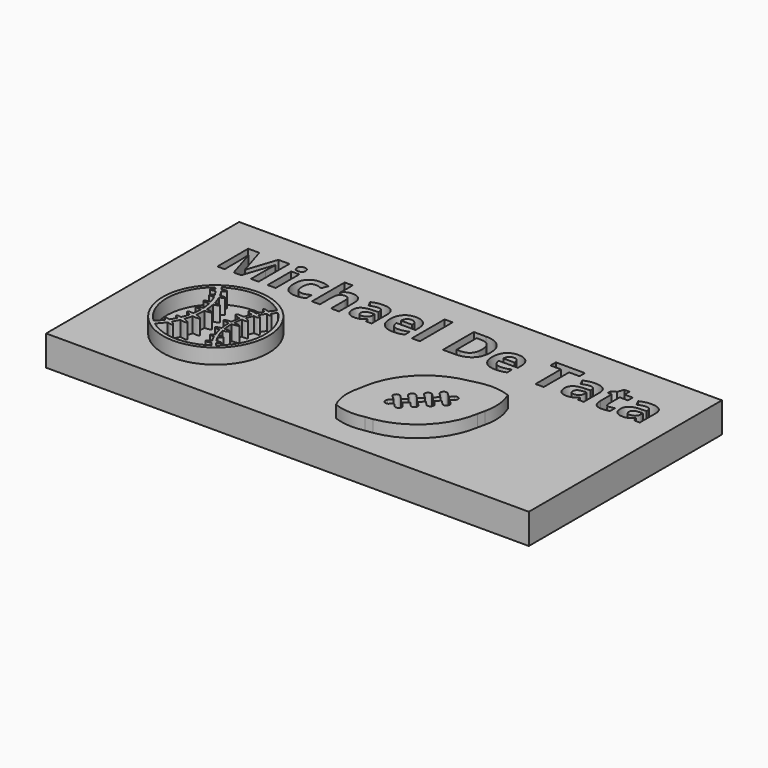
from build123d import *

# Parameters (mm, degrees)
F0_W         = 101.6
F0_H         = 50.8
F1_DEPTH     = 6.35
F3_R         = 11.1218952469
F4_DEPTH     = 3.175
F6_DEPTH     = 2.54
F2_TEXT_SIZE = 11.3601718719
F7_DEPTH     = 3.175


# Not quite as in the source:
# - a feature names something its author has since deleted; it is built from what else it names
# - Text() gives the source's letters only with a copy of the font that has no kerning and outlines rounded to 1/6400 em; it was checked with that copy


with BuildPart() as f1:
    # F0 (on Top) → F1 (new body)
    with BuildSketch(Plane.XY):
        Rectangle(F0_W, F0_H)
    extrude(amount=F1_DEPTH)

    # F3 (on face) → F4 (join)
    with BuildSketch(Plane.XY.offset(6.35)):
        with Locations((-29.0186479688, -7.998152636)):
            Circle(F3_R)
        with BuildLine():
            ThreePointArc((-22.6005740509, -1.5785002837), (-22.1799453907, -1.1150611958), (-21.7337125174, -0.6762212695))
            ThreePointArc((-21.7337125174, -0.6762212695), (-18.7036022056, -8.5280529742), (-22.5223602891, -16.0280473955))
            ThreePointArc((-22.5223602891, -16.0280473955), (-22.7780684113, -15.7253880437), (-23.0227432081, -15.4137414958))
            add(Edge.make_bspline(
                [(-23.0227432081, -15.4137414958), (-19.8096573759, -13.5154492667), (-23.4284209645, -14.8404104762)],
                knots=[5.0949228166, 5.0949228166, 5.0949228166, 7.5723181465, 7.5723181465, 7.5723181465], degree=2, weights=[1, 0.3260277363, 1]))
            ThreePointArc((-23.4284209645, -14.8404104762), (-23.805157256, -14.2278051435), (-24.1411783748, -13.5919550552))
            add(Edge.make_bspline(
                [(-24.1411783748, -13.5919550552), (-23.230493802, -13.2932672954), (-23.3456804393, -13.0374149632), (-23.4608670766, -12.7815626311), (-24.417649348, -12.9778582733)],
                knots=[4.9642155268, 4.9642155268, 4.9642155268, 6.3335518412, 6.3335518412, 7.7028881555, 7.7028881555, 7.7028881555], degree=2, weights=[1, 0.7746289525, 1, 0.7746289525, 1]))
            ThreePointArc((-24.417649348, -12.9778582733), (-24.7272451793, -12.1343360676), (-24.9671670987, -11.2684164623))
            add(Edge.make_bspline(
                [(-24.9671670987, -11.2684164623), (-23.7185142099, -11.0757901304), (-23.7819942791, -10.7558740683), (-23.8454743483, -10.4359580061), (-25.1117428322, -10.5398082556)],
                knots=[4.8729813766, 4.8729813766, 4.8729813766, 6.3045795957, 6.3045795957, 7.7361778148, 7.7361778148, 7.7361778148], degree=2, weights=[1, 0.75456909, 1, 0.75456909, 1]))
            ThreePointArc((-25.1117428322, -10.5398082556), (-25.2292975786, -9.5332747384), (-25.2539958206, -8.5202007843))
            add(Edge.make_bspline(
                [(-25.2539958206, -8.5202007843), (-23.9044438188, -8.4744131194), (-23.8901319743, -8.1956421106), (-23.8758201297, -7.9168711017), (-25.2203758909, -7.8653402803)],
                knots=[4.8773757852, 4.8773757852, 4.8773757852, 6.2727242396, 6.2727242396, 7.6680726941, 7.6680726941, 7.6680726941], degree=2, weights=[1, 0.7663384213, 1, 0.7663384213, 1]))
            ThreePointArc((-25.2203758909, -7.8653402803), (-25.1208078752, -7.0327925831), (-24.9582957446, -6.2102117269))
            add(Edge.make_bspline(
                [(-24.9582957446, -6.2102117269), (-20.6595931309, -6.796804342), (-24.7459385815, -5.4406721979)],
                knots=[5.0315591498, 5.0315591498, 5.0315591498, 7.5106380767, 7.5106380767, 7.5106380767], degree=2, weights=[1, 0.3252318181, 1]))
            ThreePointArc((-24.7459385815, -5.4406721979), (-24.4822237672, -4.6979294002), (-24.1661512275, -3.9759110372))
            add(Edge.make_bspline(
                [(-24.1661512275, -3.9759110372), (-20.9222938258, -4.6172431349), (-23.7986605821, -3.2771255195)],
                knots=[5.0646772946, 5.0646772946, 5.0646772946, 7.3959785173, 7.3959785173, 7.3959785173], degree=2, weights=[1, 0.3941526836, 1]))
            ThreePointArc((-23.7986605821, -3.2771255195), (-23.4215564836, -2.6655092164), (-23.0054379696, -2.0797384545))
            add(Edge.make_bspline(
                [(-23.0054379696, -2.0797384545), (-20.3352108354, -2.919747127), (-22.6005740509, -1.5785002837)],
                knots=[5.0589564234, 5.0589564234, 5.0589564234, 7.3589787004, 7.3589787004, 7.3589787004], degree=2, weights=[1, 0.408477274, 1]))
        make_face(mode=Mode.SUBTRACT)
        with BuildLine():
            ThreePointArc((-36.0519275049, -15.5621424847), (-39.3420122611, -7.6678298334), (-35.5539764132, 0))
            ThreePointArc((-35.5539764132, 0), (-35.35460765, -0.2062619443), (-35.1608345722, -0.4177894547))
            add(Edge.make_bspline(
                [(-35.1608345722, -0.4177894547), (-37.7982757436, -2.1762355745), (-34.7023311185, -0.9679386151)],
                knots=[2.0229375925, 2.0229375925, 2.0229375925, 4.3852414284, 4.3852414284, 4.3852414284], degree=2, weights=[1, 0.3798595016, 1]))
            ThreePointArc((-34.7023311185, -0.9679386151), (-34.2949359087, -1.527849727), (-33.9245732543, -2.1129162313))
            add(Edge.make_bspline(
                [(-33.9245732543, -2.1129162313), (-37.2277823305, -3.6536940562), (-33.5874672551, -2.7312571551)],
                knots=[1.9552328248, 1.9552328248, 1.9552328248, 4.4201232192, 4.4201232192, 4.4201232192], degree=2, weights=[1, 0.3319321592, 1]))
            ThreePointArc((-33.5874672551, -2.7312571551), (-33.2140250787, -3.5589351008), (-32.9120345986, -4.4152712444))
            add(Edge.make_bspline(
                [(-32.9120345986, -4.4152712444), (-34.1483285306, -4.6541693743), (-34.0707584589, -4.9420653759), (-33.9931883873, -5.2299613774), (-32.7256886081, -5.1068816097)],
                knots=[1.8023954855, 1.8023954855, 1.8023954855, 3.170663936, 3.170663936, 4.5389323865, 4.5389323865, 4.5389323865], degree=2, weights=[1, 0.7749665091, 1, 0.7749665091, 1]))
            ThreePointArc((-32.7256886081, -5.1068816097), (-32.5525243736, -6.0270238287), (-32.4603856609, -6.958773802))
            add(Edge.make_bspline(
                [(-32.4603856609, -6.958773802), (-33.8480769362, -7.0137831609), (-33.8414401354, -7.2896008469), (-33.8348033345, -7.5654185328), (-32.4445257743, -7.6178921517)],
                knots=[1.7715815328, 1.7715815328, 1.7715815328, 3.1462792098, 3.1462792098, 4.5209768868, 4.5209768868, 4.5209768868], degree=2, weights=[1, 0.7729308655, 1, 0.7729308655, 1]))
            ThreePointArc((-32.4445257743, -7.6178921517), (-32.488635289, -8.5195254569), (-32.6085160069, -9.4142415458))
            add(Edge.make_bspline(
                [(-32.6085160069, -9.4142415458), (-36.9972444639, -8.8518803338), (-32.7586754015, -10.1217847591)],
                knots=[1.9033850235, 1.9033850235, 1.9033850235, 4.379874232, 4.379874232, 4.379874232], degree=2, weights=[1, 0.3264560084, 1]))
            ThreePointArc((-32.7586754015, -10.1217847591), (-32.9938018326, -10.9324023236), (-33.2920310018, -11.721987428))
            add(Edge.make_bspline(
                [(-33.2920310018, -11.721987428), (-36.1690854529, -11.2401260388), (-33.5703416762, -12.3262507069)],
                knots=[1.9795308567, 1.9795308567, 1.9795308567, 4.2252146249, 4.2252146249, 4.2252146249], degree=2, weights=[1, 0.4331227092, 1]))
            ThreePointArc((-33.5703416762, -12.3262507069), (-33.9150089726, -12.9624918103), (-34.3018512886, -13.5740073942))
            add(Edge.make_bspline(
                [(-34.3018512886, -13.5740073942), (-36.7715845297, -12.7356918477), (-34.7165123024, -14.1419316901)],
                knots=[1.9598946097, 1.9598946097, 1.9598946097, 4.2150352925, 4.2150352925, 4.2150352925], degree=2, weights=[1, 0.4288559593, 1]))
            ThreePointArc((-34.7165123024, -14.1419316901), (-35.3518393665, -14.8824843011), (-36.0519275049, -15.5621424847))
        make_face(mode=Mode.SUBTRACT)
        with BuildLine():
            ThreePointArc((-23.1383760068, -16.4895226738), (-29.2362070327, -18.3245087948), (-35.2513412418, -16.2343227429))
            ThreePointArc((-35.2513412418, -16.2343227429), (-34.5366397343, -15.4339446067), (-33.8932233713, -14.5752136886))
            add(Edge.make_bspline(
                [(-33.8932233713, -14.5752136886), (-32.9665372675, -14.9444901641), (-32.8065086025, -14.6949646645), (-32.6464799375, -14.4454391649), (-33.4906960246, -13.9475709017)],
                knots=[4.9366840342, 4.9366840342, 4.9366840342, 6.2468676323, 6.2468676323, 7.5570512303, 7.5570512303, 7.5570512303], degree=2, weights=[1, 0.7929920045, 1, 0.7929920045, 1]))
            ThreePointArc((-33.4906960246, -13.9475709017), (-33.1163152353, -13.277835473), (-32.7837347826, -12.5863900577))
            add(Edge.make_bspline(
                [(-32.7837347826, -12.5863900577), (-31.4628142379, -12.9251957543), (-31.3377454507, -12.6195670965), (-31.2126766634, -12.3139384387), (-32.5073316229, -11.9109479388)],
                knots=[4.7889246183, 4.7889246183, 4.7889246183, 6.254522462, 6.254522462, 7.7201203058, 7.7201203058, 7.7201203058], degree=2, weights=[1, 0.7433049699, 1, 0.7433049699, 1]))
            ThreePointArc((-32.5073316229, -11.9109479388), (-32.2375308957, -11.1114599941), (-32.0222881236, -10.295589934))
            add(Edge.make_bspline(
                [(-32.0222881236, -10.295589934), (-30.6566290985, -10.537023699), (-30.5925615236, -10.2106892216), (-30.5284939486, -9.8843547442), (-31.8762920845, -9.5519447883)],
                knots=[4.8558971312, 4.8558971312, 4.8558971312, 6.2868470545, 6.2868470545, 7.7177969778, 7.7177969778, 7.7177969778], degree=2, weights=[1, 0.7547817629, 1, 0.7547817629, 1]))
            ThreePointArc((-31.8762920845, -9.5519447883), (-31.7553675058, -8.58649868), (-31.7099105477, -7.6145714159))
            add(Edge.make_bspline(
                [(-31.7099105477, -7.6145714159), (-30.3863376738, -7.5520804997), (-30.3912068146, -7.2868248678), (-30.3960759554, -7.0215692359), (-31.7219091808, -6.960923237)],
                knots=[4.9502104898, 4.9502104898, 4.9502104898, 6.2867605554, 6.2867605554, 7.623310621, 7.623310621, 7.623310621], degree=2, weights=[1, 0.7848916797, 1, 0.7848916797, 1]))
            ThreePointArc((-31.7219091808, -6.960923237), (-31.8055927228, -5.9704302032), (-31.9677240792, -4.9897198441))
            add(Edge.make_bspline(
                [(-31.9677240792, -4.9897198441), (-27.1125520616, -3.9453633133), (-32.1277186275, -4.3110286982)],
                knots=[5.029190786, 5.029190786, 5.029190786, 7.5806409095, 7.5806409095, 7.5806409095], degree=2, weights=[1, 0.2908080359, 1]))
            ThreePointArc((-32.1277186275, -4.3110286982), (-32.4182256939, -3.3681910181), (-32.7821929472, -2.451204058))
            add(Edge.make_bspline(
                [(-32.7821929472, -2.451204058), (-29.0274258726, -0.7635566453), (-33.0867657916, -1.8135372071)],
                knots=[5.0504879678, 5.0504879678, 5.0504879678, 7.5788223687, 7.5788223687, 7.5788223687], degree=2, weights=[1, 0.3018467132, 1]))
            ThreePointArc((-33.0867657916, -1.8135372071), (-33.4449253366, -1.163453471), (-33.841041062, -0.5357756431))
            add(Edge.make_bspline(
                [(-33.841041062, -0.5357756431), (-30.3251283572, 1.6633700745), (-34.2639978839, 0.0545364371)],
                knots=[5.0699205856, 5.0699205856, 5.0699205856, 7.5815862515, 7.5815862515, 7.5815862515], degree=2, weights=[1, 0.3097817611, 1]))
            ThreePointArc((-34.2639978839, 0.0545364371), (-34.4867682203, 0.33850786), (-34.7176451358, 0.6159285545))
            ThreePointArc((-34.7176451358, 0.6159285545), (-28.4482874146, 2.3147350442), (-22.4044991055, -0.0650575098))
            ThreePointArc((-22.4044991055, -0.0650575098), (-22.9008944199, -0.6279311781), (-23.3630214119, -1.2192633333))
            add(Edge.make_bspline(
                [(-23.3630214119, -1.2192633333), (-24.3519505665, -0.8519993652), (-24.5112814604, -1.0814969003), (-24.6706123543, -1.3109944355), (-23.7496992537, -1.7762275822)],
                knots=[1.7313775886, 1.7313775886, 1.7313775886, 3.0870763276, 3.0870763276, 4.4427750666, 4.4427750666, 4.4427750666], degree=2, weights=[1, 0.7789232209, 1, 0.7789232209, 1]))
            ThreePointArc((-23.7496992537, -1.7762275822), (-24.1276414609, -2.3905663915), (-24.4699386242, -3.0254562533))
            add(Edge.make_bspline(
                [(-24.4699386242, -3.0254562533), (-25.8098987721, -2.6275472634), (-25.9760824588, -2.9876997869), (-26.1422661455, -3.3478523104), (-24.8261870356, -3.7975161764)],
                knots=[1.6047845986, 1.6047845986, 1.6047845986, 3.1036676273, 3.1036676273, 4.6025506559, 4.6025506559, 4.6025506559], degree=2, weights=[1, 0.7320694402, 1, 0.7320694402, 1]))
            ThreePointArc((-24.8261870356, -3.7975161764), (-25.1084652464, -4.5304584752), (-25.3446931734, -5.2795123906))
            add(Edge.make_bspline(
                [(-25.3446931734, -5.2795123906), (-26.7791841224, -4.97609655), (-26.8736810972, -5.3603493644), (-26.968178072, -5.7446021788), (-25.5457240749, -6.0969638472)],
                knots=[1.6300234577, 1.6300234577, 1.6300234577, 3.1370870325, 3.1370870325, 4.6441506072, 4.6441506072, 4.6441506072], degree=2, weights=[1, 0.7292769073, 1, 0.7292769073, 1]))
            ThreePointArc((-25.5457240749, -6.0969638472), (-25.6989600987, -6.9762304815), (-25.7897887641, -7.8641163112))
            add(Edge.make_bspline(
                [(-25.7897887641, -7.8641163112), (-27.1425839364, -7.9099645752), (-27.1539666106, -8.1894030613), (-27.1653492847, -8.4688415473), (-25.816475426, -8.5192594086)],
                knots=[1.7356086307, 1.7356086307, 1.7356086307, 3.1332923886, 3.1332923886, 4.5309761466, 4.5309761466, 4.5309761466], degree=2, weights=[1, 0.7655877563, 1, 0.7655877563, 1]))
            ThreePointArc((-25.816475426, -8.5192594086), (-25.788340047, -9.569604801), (-25.6730954344, -10.6139877395))
            add(Edge.make_bspline(
                [(-25.6730954344, -10.6139877395), (-26.7543096913, -10.8133630796), (-26.7023555836, -11.0986327553), (-26.650401476, -11.383902431), (-25.5431388197, -11.3275536729)],
                knots=[1.841558468, 1.841558468, 1.841558468, 3.1589653359, 3.1589653359, 4.4763722037, 4.4763722037, 4.4763722037], degree=2, weights=[1, 0.7907865138, 1, 0.7907865138, 1]))
            ThreePointArc((-25.5431388197, -11.3275536729), (-25.3120149888, -12.2467944829), (-25.0126804516, -13.1461390926))
            add(Edge.make_bspline(
                [(-25.0126804516, -13.1461390926), (-28.1227231988, -14.2915891351), (-24.7702075678, -13.7456005418)],
                knots=[1.9398124101, 1.9398124101, 1.9398124101, 4.4219337452, 4.4219337452, 4.4219337452], degree=2, weights=[1, 0.3237929395, 1]))
            ThreePointArc((-24.7702075678, -13.7456005418), (-24.439671853, -14.4466246637), (-24.0668076782, -15.1260810533))
            add(Edge.make_bspline(
                [(-24.0668076782, -15.1260810533), (-25.0420902547, -15.6459049386), (-24.8810492506, -15.902122303), (-24.7200082464, -16.1583396673), (-23.6821681389, -15.7380452517)],
                knots=[1.801867732, 1.801867732, 1.801867732, 3.1771930657, 3.1771930657, 4.5525183994, 4.5525183994, 4.5525183994], degree=2, weights=[1, 0.7727317064, 1, 0.7727317064, 1]))
            ThreePointArc((-23.6821681389, -15.7380452517), (-23.4171654624, -16.1187722311), (-23.1383760068, -16.4895226738))
        make_face(mode=Mode.SUBTRACT)
    extrude(amount=F4_DEPTH)

    # F5 (on face) → F6 (join)
    with BuildSketch(Plane.XY.offset(6.35)):
        with BuildLine():
            ThreePointArc((4.5972601511, -12.5120617449), (4.3143412648, -15.9226333064), (5.2721370012, -19.2081574351))
            ThreePointArc((5.2721370012, -19.2081574351), (8.4792166768, -19.9150856323), (11.7527060211, -19.6516942233))
            Line((11.7527060211, -19.6516942233), (13.2659822702, -19.4572750479))
            ThreePointArc((13.2659822702, -19.4572750479), (21.3262171238, -15.3390412719), (25.4755634815, -7.2947787121))
            Line((25.4755634815, -7.2947787121), (25.8165318519, -5.7179266587))
            ThreePointArc((25.8165318519, -5.7179266587), (26.0664069713, -2.2732548821), (25.1938384026, 1.068425132))
            ThreePointArc((25.1938384026, 1.068425132), (21.9865075076, 1.7577248565), (18.7178328633, 1.4786699321))
            Line((18.7178328633, 1.4786699321), (17.0773006976, 1.068425132))
            ThreePointArc((17.0773006976, 1.068425132), (9.0415260088, -3.0197044149), (4.867607262, -11.0112549737))
            Line((4.867607262, -11.0112549737), (4.5972601511, -12.5120617449))
        make_face()
        with BuildLine():
            Line((17.1466153115, -4.6676485799), (18.0364530534, -5.4857870564))
            Line((18.0364530534, -5.4857870564), (18.7178328633, -4.8015508705))
            ThreePointArc((18.7178328633, -4.8015508705), (19.5414278726, -4.7701809468), (19.6319296956, -5.5893892422))
            Line((19.6319296956, -5.5893892422), (18.906712532, -6.339806132))
            Line((18.906712532, -6.339806132), (19.8530521194, -7.2543667192))
            ThreePointArc((19.8530521194, -7.2543667192), (19.7318680066, -8.0693349588), (18.9323183149, -8.2682799548))
            Line((18.9323183149, -8.2682799548), (17.9688166827, -7.273696363))
            Line((17.9688166827, -7.273696363), (17.0569783471, -8.15703863))
            Line((17.0569783471, -8.15703863), (17.9408057089, -9.0693777093))
            ThreePointArc((17.9408057089, -9.0693777093), (17.9026988116, -9.9087533416), (17.0892104506, -10.1190870628))
            Line((17.0892104506, -10.1190870628), (16.1368567497, -9.1667333618))
            Line((16.1368567497, -9.1667333618), (15.1845030487, -10.1190870628))
            Line((15.1845030487, -10.1190870628), (15.9585415386, -10.8931255527))
            ThreePointArc((15.9585415386, -10.8931255527), (16.003442938, -11.7581809417), (15.1476850733, -11.8924025446))
            Line((15.1476850733, -11.8924025446), (14.3097722903, -10.9931109473))
            Line((14.3097722903, -10.9931109473), (13.3446057558, -11.8924025446))
            Line((13.3446057558, -11.8924025446), (14.1482524708, -12.7549180148))
            ThreePointArc((14.1482524708, -12.7549180148), (14.1061184062, -13.6956929178), (13.1663065404, -13.6358067393))
            Line((13.1663065404, -13.6358067393), (12.4410521239, -12.8885759041))
            Line((12.4410521239, -12.8885759041), (11.8110338226, -13.6358067393))
            ThreePointArc((11.8110338226, -13.6358067393), (10.9103253637, -13.493421619), (10.8000738546, -12.5882178545))
            Line((10.8000738546, -12.5882178545), (11.5428594872, -11.9029218331))
            Line((11.5428594872, -11.9029218331), (10.550509207, -11.0182818025))
            ThreePointArc((10.550509207, -11.0182818025), (10.6959906178, -10.1732211816), (11.5523757413, -10.1296687499))
            Line((11.5523757413, -10.1296687499), (12.4061414972, -11.0008576885))
            Line((12.4061414972, -11.0008576885), (13.2951091813, -10.1296687499))
            Line((13.2951091813, -10.1296687499), (12.3939610977, -9.210130531))
            ThreePointArc((12.3939610977, -9.210130531), (12.5566341915, -8.3211622257), (13.4602803737, -8.3088837564))
            Line((13.4602803737, -8.3088837564), (14.2704863101, -9.1539369896))
            Line((14.2704863101, -9.1539369896), (15.2218611187, -8.24179384))
            Line((15.2218611187, -8.24179384), (14.237829484, -7.330563385))
            ThreePointArc((14.237829484, -7.330563385), (14.4077394845, -6.4651482984), (15.2891669422, -6.4351763576))
            Line((15.2891669422, -6.4351763576), (16.097266227, -7.2847162373))
            Line((16.097266227, -7.2847162373), (16.9903718402, -6.4351763576))
            Line((16.9903718402, -6.4351763576), (16.1511966242, -5.5529669244))
            ThreePointArc((16.1511966242, -5.5529669244), (16.1911729289, -4.5956499191), (17.1466153115, -4.6676485799))
        make_face(mode=Mode.SUBTRACT)
    extrude(amount=F6_DEPTH)

    # F2 (on face) → F7 (cut)
    with BuildSketch(Plane.XY.offset(6.35)):
        with Locations((-44.7246991098, 10.7928151265)):
            Text('Michael De Tata', F2_TEXT_SIZE, font='Open Sans', font_style=FontStyle.BOLD, text_align=(TextAlign.LEFT, TextAlign.BOTTOM))
    extrude(amount=-F7_DEPTH, mode=Mode.SUBTRACT)


solid = f1.part
